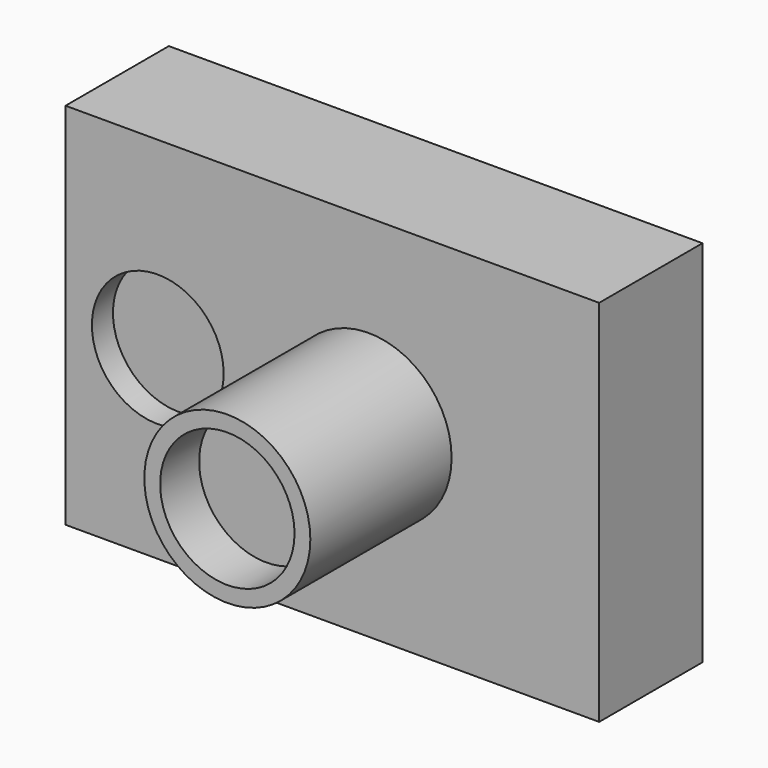
from build123d import *

# Parameters (mm, degrees)
F0_W     = 40.5
F0_H     = 28
F1_DEPTH = 9.8
F2_R     = 6.3
F2_R_2   = 5.1
F3_DEPTH = 13.4
F4_DEPTH = 9.7
F5_R     = 5
F6_DEPTH = 2


# Not quite as in the source:
# - a feature of the source that left no trace in its solid (it failed there, or was rolled back) is left out


with BuildPart() as f1:
    # F0 (on Front) → F1 (new body)
    with BuildSketch(Plane.XZ):
        with Locations((20.25, -14)):
            Rectangle(F0_W, F0_H)
    extrude(amount=F1_DEPTH)

    # F2 (on face) → F3 (join)
    with BuildSketch(Plane.XZ.offset(9.8)):
        with Locations((23, -14)):
            Circle(F2_R)
        with Locations((23, -14)):
            Circle(F2_R_2, mode=Mode.SUBTRACT)
    extrude(amount=F3_DEPTH)

    # F4 (add): a face of the model
    f4_faces = [f1.faces().sort_by_distance(p)[0] for p in [
        (23, -9.8, -14),
    ]]
    extrude(f4_faces, amount=F4_DEPTH)

    # F5 (on face) → F6 (cut)
    with BuildSketch(Plane.XZ.offset(9.8)):
        with Locations((7, -14)):
            Circle(F5_R)
    extrude(amount=-F6_DEPTH, mode=Mode.SUBTRACT)


solid = f1.part
